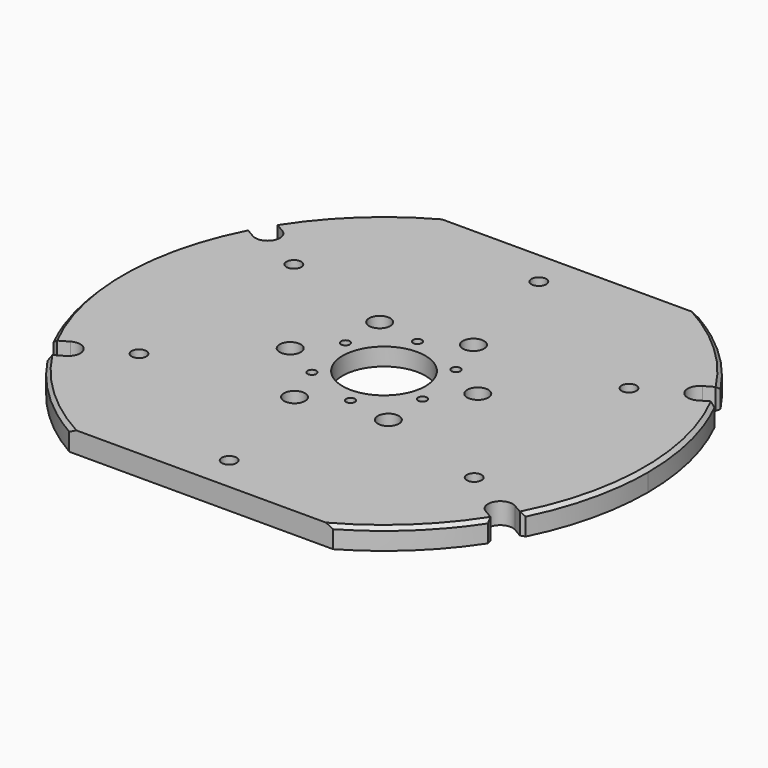
from build123d import *

# Parameters (mm, degrees)
F0_R          = 4.2
F0_R_2        = 23.5
F1_DEPTH      = 12
F3_R          = 40
F4_DEPTH      = 2
F4_DEPTH_BACK = 10
F6_D          = 5
F7_D          = 12
F9_T1_DEPTH   = 22.4125042877
F9_T4_ANGLE   = 31.2546131469
F9_T6_ANGLE   = 58.580275092
F9_T8_ANGLE   = 31.2546131469
F9_T10_ANGLE  = 31.2546131469
F9_T12_ANGLE  = 58.580275092
F9_T14_ANGLE  = 31.2546131469


# Not quite as in the source:
# - a fillet or chamfer that OpenCascade refuses, or shapes differently, is made with other operations: its cross-section is extruded or revolved along the edge and cut away or added
# - a feature of the source that left no trace in its solid (it failed there, or was rolled back) is left out


with BuildPart() as f1:
    # F0 (on Top) → F1 (new body)
    with BuildSketch(Plane.XY):
        with BuildLine():
            Line((75, 129.9038105677), (-75, 129.9038105677))
            ThreePointArc((-75, 129.9038105677), (-103.561575886, 108.5126720711), (-126.2622826556, 80.9804666484))
            Line((-126.2622826556, 80.9804666484), (-119.3923048454, 77.0140831103))
            ThreePointArc((-119.3923048454, 77.0140831103), (-116.8301270189, 67.4519052838), (-126.3923048454, 64.8897274573))
            Line((-126.3923048454, 64.8897274573), (-133.2622826556, 68.8561109954))
            ThreePointArc((-133.2622826556, 68.8561109954), (-145.7555185891, 35.4306195377), (-150, 0))
            ThreePointArc((-150, 0), (-145.7555185891, -35.4306195377), (-133.2622826556, -68.8561109954))
            Line((-133.2622826556, -68.8561109954), (-126.3923048454, -64.8897274573))
            ThreePointArc((-126.3923048454, -64.8897274573), (-116.8301270189, -67.4519052838), (-119.3923048454, -77.0140831103))
            Line((-119.3923048454, -77.0140831103), (-126.2622826556, -80.9804666484))
            ThreePointArc((-126.2622826556, -80.9804666484), (-103.561575886, -108.5126720711), (-75, -129.9038105677))
            Line((-75, -129.9038105677), (75, -129.9038105677))
            ThreePointArc((75, -129.9038105677), (103.561575886, -108.5126720711), (126.2622826556, -80.9804666484))
            Line((126.2622826556, -80.9804666484), (119.3923048454, -77.0140831103))
            ThreePointArc((119.3923048454, -77.0140831103), (116.8301270189, -67.4519052838), (126.3923048454, -64.8897274573))
            Line((126.3923048454, -64.8897274573), (133.2622826556, -68.8561109954))
            ThreePointArc((133.2622826556, -68.8561109954), (145.7555185891, -35.4306195377), (150, 0))
            ThreePointArc((150, 0), (145.7555185891, 35.4306195377), (133.2622826556, 68.8561109954))
            Line((133.2622826556, 68.8561109954), (126.3923048454, 64.8897274573))
            ThreePointArc((126.3923048454, 64.8897274573), (116.8301270189, 67.4519052838), (119.3923048454, 77.0140831103))
            Line((119.3923048454, 77.0140831103), (126.2622826556, 80.9804666484))
            ThreePointArc((126.2622826556, 80.9804666484), (103.561575886, 108.5126720711), (75, 129.9038105677))
        make_face()
        with Locations((-95.2627944163, -55)):
            Circle(F0_R, mode=Mode.SUBTRACT)
        with Locations((0, -110)):
            Circle(F0_R, mode=Mode.SUBTRACT)
        with Locations((95.2627944163, -55)):
            Circle(F0_R, mode=Mode.SUBTRACT)
        with Locations((-95.2627944163, 55)):
            Circle(F0_R, mode=Mode.SUBTRACT)
        Circle(F0_R_2, mode=Mode.SUBTRACT)
        with Locations((95.2627944163, 55)):
            Circle(F0_R, mode=Mode.SUBTRACT)
        with Locations((0, 110)):
            Circle(F0_R, mode=Mode.SUBTRACT)
    extrude(amount=-F1_DEPTH)

    # F3 (on offset) → F4 (cut, two sides)
    with BuildSketch(Plane(origin=(0, 0, -12), x_dir=(1, 0, 0), z_dir=(0, 0, -1))) as f4_sk:
        Circle(F3_R)
    extrude(amount=-F4_DEPTH, mode=Mode.SUBTRACT)
    extrude(f4_sk.sketch, amount=F4_DEPTH_BACK, mode=Mode.SUBTRACT)

    # F6 (through all)
    with Locations(Plane(origin=(0, 0, -12), x_dir=(1, 0, 0), z_dir=(0, 0, -1))):
        with Locations((6.105887852, 31.4120698703), (-24.1507065671, 20.9938889277), (-30.2565944192, -10.4181809426), (-6.105887852, -31.4120698703), (24.1507065671, -20.9938889277), (30.2565944192, 10.4181809426)):
            Hole(F6_D / 2)

    # F7 (through all)
    with Locations(Plane(origin=(0, 0, -12), x_dir=(1, 0, 0), z_dir=(0, 0, -1))):
        with Locations((-30.8347743626, -35.4713502705), (15.3017032595, -44.4393730532), (46.136477622, -8.9680227827), (30.8347743626, 35.4713502705), (-15.3017032595, 44.4393730532), (-46.136477622, 8.9680227827)):
            Hole(F7_D / 2)

    # F9: chamfer of 2 on 14 edges, made by hand

    # F9_s2 → F9_t1 (cut)
    with BuildSketch(Plane.XY.offset(-17.2062521438)):
        with BuildLine():
            Line((124.5001445289, -79.8958399675), (125.1751296186, -82.7566727445))
            Line((125.1751296186, -82.7566727445), (125.2085047543, -82.7787204273))
            ThreePointArc((125.2085047543, -82.7787204273), (125.7308425606, -81.8764729883), (126.2959525977, -81.0020614395))
            Line((126.2959525977, -81.0020614395), (126.2822826556, -80.9458256322))
            ThreePointArc((126.2822826556, -80.9458256322), (125.3866522933, -80.4287332014), (124.5201445289, -79.8611989514))
            Line((124.5201445289, -79.8611989514), (124.5001445289, -79.8958399675))
        make_face()
        with BuildLine():
            Line((131.441899333, -67.8723679531), (134.2569457387, -67.0265057995))
            Line((134.2569457387, -67.0265057995), (134.29272716, -67.0443856735))
            ThreePointArc((134.29272716, -67.0443856735), (133.7725268604, -67.9478672025), (133.2978192643, -68.874472625))
            Line((133.2978192643, -68.874472625), (133.2422826556, -68.8907520115))
            ThreePointArc((133.2422826556, -68.8907520115), (132.3466522933, -68.3736595808), (131.421899333, -67.9070089693))
            Line((131.421899333, -67.9070089693), (131.441899333, -67.8723679531))
        make_face()
        with BuildLine():
            Line((-125.1751296186, -82.7566727445), (-124.5001445289, -79.8958399675))
            Line((-124.5001445289, -79.8958399675), (-124.5201445289, -79.8611989514))
            ThreePointArc((-124.5201445289, -79.8611989514), (-125.3866522933, -80.4287332014), (-126.2822826556, -80.9458256322))
            Line((-126.2822826556, -80.9458256322), (-126.2959525977, -81.0020614395))
            ThreePointArc((-126.2959525977, -81.0020614395), (-125.7308425606, -81.8764729883), (-125.2085047543, -82.7787204273))
            Line((-125.2085047543, -82.7787204273), (-125.1751296186, -82.7566727445))
        make_face()
        with BuildLine():
            Line((134.2569457387, 67.0265057995), (131.441899333, 67.8723679531))
            Line((131.441899333, 67.8723679531), (131.421899333, 67.9070089693))
            ThreePointArc((131.421899333, 67.9070089693), (132.3466522933, 68.3736595808), (133.2422826556, 68.8907520115))
            Line((133.2422826556, 68.8907520115), (133.2978192643, 68.874472625))
            ThreePointArc((133.2978192643, 68.874472625), (133.7725268604, 67.9478672025), (134.29272716, 67.0443856735))
            Line((134.29272716, 67.0443856735), (134.2569457387, 67.0265057995))
        make_face()
        with BuildLine():
            Line((-131.441899333, -67.8723679531), (-134.2569457387, -67.0265057995))
            Line((-134.2569457387, -67.0265057995), (-134.29272716, -67.0443856735))
            ThreePointArc((-134.29272716, -67.0443856735), (-133.7725268604, -67.9478672025), (-133.2978192643, -68.874472625))
            Line((-133.2978192643, -68.874472625), (-133.2422826556, -68.8907520115))
            ThreePointArc((-133.2422826556, -68.8907520115), (-132.3466522933, -68.3736595808), (-131.421899333, -67.9070089693))
            Line((-131.421899333, -67.9070089693), (-131.441899333, -67.8723679531))
        make_face()
        with BuildLine():
            Line((124.5001445289, 79.8958399675), (125.1751296186, 82.7566727445))
            Line((125.1751296186, 82.7566727445), (125.2085047543, 82.7787204273))
            ThreePointArc((125.2085047543, 82.7787204273), (125.7308425606, 81.8764729883), (126.2959525977, 81.0020614395))
            Line((126.2959525977, 81.0020614395), (126.2822826556, 80.9458256322))
            ThreePointArc((126.2822826556, 80.9458256322), (125.3866522933, 80.4287332014), (124.5201445289, 79.8611989514))
            Line((124.5201445289, 79.8611989514), (124.5001445289, 79.8958399675))
        make_face()
        with BuildLine():
            Line((-134.2569457387, 67.0265057995), (-131.441899333, 67.8723679531))
            Line((-131.441899333, 67.8723679531), (-131.421899333, 67.9070089693))
            ThreePointArc((-131.421899333, 67.9070089693), (-132.3466522933, 68.3736595808), (-133.2422826556, 68.8907520115))
            Line((-133.2422826556, 68.8907520115), (-133.2978192643, 68.874472625))
            ThreePointArc((-133.2978192643, 68.874472625), (-133.7725268604, 67.9478672025), (-134.29272716, 67.0443856735))
            Line((-134.29272716, 67.0443856735), (-134.2569457387, 67.0265057995))
        make_face()
        with BuildLine():
            Line((-125.1751296186, 82.7566727445), (-124.5001445289, 79.8958399675))
            Line((-124.5001445289, 79.8958399675), (-124.5201445289, 79.8611989514))
            ThreePointArc((-124.5201445289, 79.8611989514), (-125.3866522933, 80.4287332014), (-126.2822826556, 80.9458256322))
            Line((-126.2822826556, 80.9458256322), (-126.2959525977, 81.0020614395))
            ThreePointArc((-126.2959525977, 81.0020614395), (-125.7308425606, 81.8764729883), (-125.2085047543, 82.7787204273))
            Line((-125.2085047543, 82.7787204273), (-125.1751296186, 82.7566727445))
        make_face()
    extrude(amount=F9_T1_DEPTH, mode=Mode.SUBTRACT)

    # F9_s3 → F9_t4 (revolve, cut)
    with BuildSketch(Plane(origin=(0, 0, 0), x_dir=(0, 0, 1), z_dir=(-0.8826581326, -0.470015554, 0))):
        with BuildLine():
            Line((-2.0565685425, -150.0565685425), (0.0565685425, -147.9434314575))
            Line((0.0565685425, -147.9434314575), (0.0965685425, -147.9434314575))
            ThreePointArc((0.0965685425, -147.9434314575), (0.04, -148.9717157288), (0.04, -150))
            Line((0.04, -150), (0, -150.04))
            ThreePointArc((0, -150.04), (-1.0282842712, -150.04), (-2.0565685425, -150.0965685425))
            Line((-2.0565685425, -150.0965685425), (-2.0565685425, -150.0565685425))
        make_face()
    revolve(axis=Axis((0, 0, 0), (0, 0, 1)), revolution_arc=F9_T4_ANGLE, mode=Mode.SUBTRACT)

    # F9_s5 → F9_t6 (revolve, cut)
    with BuildSketch(Plane(origin=(0, 0, 0), x_dir=(0, 0, 1), z_dir=(-0.4892323332, 0.872153498, 0))):
        with BuildLine():
            Line((0.0565685425, 147.9434314575), (-2.0565685425, 150.0565685425))
            Line((-2.0565685425, 150.0565685425), (-2.0565685425, 150.0965685425))
            ThreePointArc((-2.0565685425, 150.0965685425), (-1.0282842712, 150.04), (0, 150.04))
            Line((0, 150.04), (0.04, 150))
            ThreePointArc((0.04, 150), (0.04, 148.9717157288), (0.0965685425, 147.9434314575))
            Line((0.0965685425, 147.9434314575), (0.0565685425, 147.9434314575))
        make_face()
    revolve(axis=Axis((0, 0, 0), (0, 0, -1)), revolution_arc=F9_T6_ANGLE, mode=Mode.SUBTRACT)

    # F9_s7 → F9_t8 (revolve, cut)
    with BuildSketch(Plane(origin=(0, 0, 0), x_dir=(0, 0, 1), z_dir=(0.5106941932, -0.8597624329, 0))):
        with BuildLine():
            Line((0.0565685425, -147.9434314575), (-2.0565685425, -150.0565685425))
            Line((-2.0565685425, -150.0565685425), (-2.0565685425, -150.0965685425))
            ThreePointArc((-2.0565685425, -150.0965685425), (-1.0282842712, -150.04), (0, -150.04))
            Line((0, -150.04), (0.04, -150))
            ThreePointArc((0.04, -150), (0.04, -148.9717157288), (0.0965685425, -147.9434314575))
            Line((0.0965685425, -147.9434314575), (0.0565685425, -147.9434314575))
        make_face()
    revolve(axis=Axis((0, 0, 0), (0, 0, 1)), revolution_arc=F9_T8_ANGLE, mode=Mode.SUBTRACT)

    # F9_s9 → F9_t10 (revolve, cut)
    with BuildSketch(Plane(origin=(0, 0, 0), x_dir=(0, 0, 1), z_dir=(0.8826581326, 0.470015554, 0))):
        with BuildLine():
            Line((0.0565685425, -147.9434314575), (-2.0565685425, -150.0565685425))
            Line((-2.0565685425, -150.0565685425), (-2.0565685425, -150.0965685425))
            ThreePointArc((-2.0565685425, -150.0965685425), (-1.0282842712, -150.04), (0, -150.04))
            Line((0, -150.04), (0.04, -150))
            ThreePointArc((0.04, -150), (0.04, -148.9717157288), (0.0965685425, -147.9434314575))
            Line((0.0965685425, -147.9434314575), (0.0565685425, -147.9434314575))
        make_face()
    revolve(axis=Axis((0, 0, 0), (0, 0, 1)), revolution_arc=F9_T10_ANGLE, mode=Mode.SUBTRACT)

    # F9_s11 → F9_t12 (revolve, cut)
    with BuildSketch(Plane(origin=(0, 0, 0), x_dir=(0, 0, 1), z_dir=(0.4892323332, -0.872153498, 0))):
        with BuildLine():
            Line((0.0565685425, 147.9434314575), (-2.0565685425, 150.0565685425))
            Line((-2.0565685425, 150.0565685425), (-2.0565685425, 150.0965685425))
            ThreePointArc((-2.0565685425, 150.0965685425), (-1.0282842712, 150.04), (0, 150.04))
            Line((0, 150.04), (0.04, 150))
            ThreePointArc((0.04, 150), (0.04, 148.9717157288), (0.0965685425, 147.9434314575))
            Line((0.0965685425, 147.9434314575), (0.0565685425, 147.9434314575))
        make_face()
    revolve(axis=Axis((0, 0, 0), (0, 0, -1)), revolution_arc=F9_T12_ANGLE, mode=Mode.SUBTRACT)

    # F9_s13 → F9_t14 (revolve, cut)
    with BuildSketch(Plane(origin=(0, 0, 0), x_dir=(0, 0, 1), z_dir=(-0.5106941932, 0.8597624329, 0))):
        with BuildLine():
            Line((0.0565685425, -147.9434314575), (-2.0565685425, -150.0565685425))
            Line((-2.0565685425, -150.0565685425), (-2.0565685425, -150.0965685425))
            ThreePointArc((-2.0565685425, -150.0965685425), (-1.0282842712, -150.04), (0, -150.04))
            Line((0, -150.04), (0.04, -150))
            ThreePointArc((0.04, -150), (0.04, -148.9717157288), (0.0965685425, -147.9434314575))
            Line((0.0965685425, -147.9434314575), (0.0565685425, -147.9434314575))
        make_face()
    revolve(axis=Axis((0, 0, 0), (0, 0, 1)), revolution_arc=F9_T14_ANGLE, mode=Mode.SUBTRACT)


solid = f1.part
